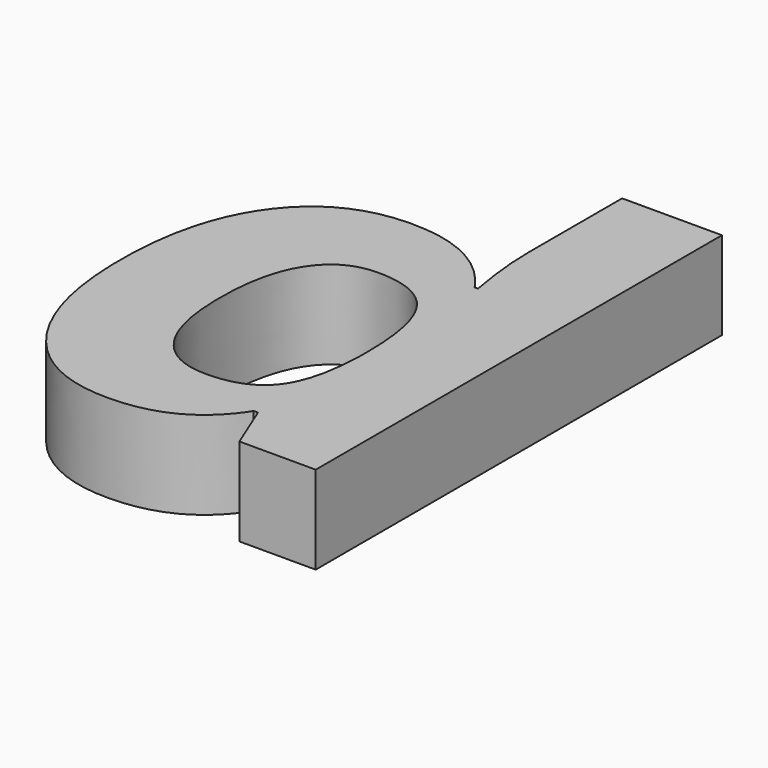
from build123d import *

# Parameters (mm, degrees)
F0_TEXT_SIZE = 75.9123669316
F1_DEPTH     = 10


# Not quite as in the source:
# - Text() gives the source's letters only with a copy of the font that has no kerning and outlines rounded to 1/6400 em; it was checked with that copy


with BuildPart() as f1:
    # F0 (on Top) → F1 (new body)
    with BuildSketch(Plane.XY):
        with Locations((0, 0)):
            Text('d', F0_TEXT_SIZE, font='Open Sans', font_style=FontStyle.BOLD, text_align=(TextAlign.LEFT, TextAlign.BOTTOM))
    extrude(amount=F1_DEPTH)


solid = f1.part
